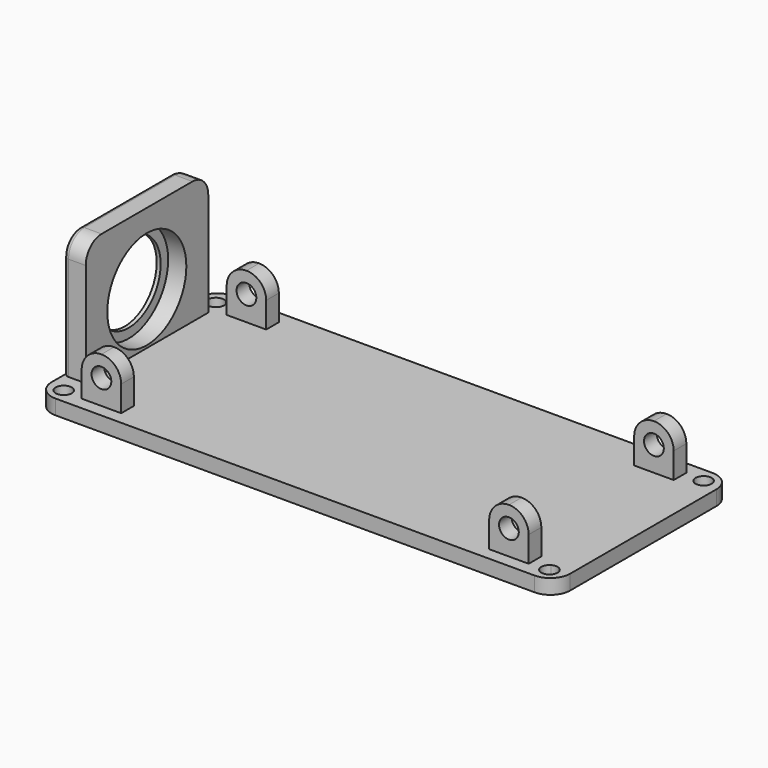
from build123d import *

# Parameters (mm, degrees)
F0_W      = 133.35
F0_H      = 57.15
F0_W_2    = 94.615
F0_H_2    = 4.064
F0_W_3    = 10.16
F0_H_3    = 42.545
F1_DEPTH  = 3.81
F2_W      = 5.6896
F2_H      = 39.37
F3_DEPTH  = 31.75
F4_R      = 5.08
F5_R      = 10.287
F6_DEPTH  = 25.4
F7_R      = 2.0701
F8_DEPTH  = 3.811
F9_R      = 5.08
F10_R     = 1.27
F11_R     = 12.7
F11_R_2   = 10.287
F12_DEPTH = 4.6736
F13_DEPTH = 15.494
F14_R     = 2.54
F15_DEPTH = 5.08
F16_R     = 2.54
F17_DEPTH = 25.4
F18_R     = 2.54
F19_DEPTH = 25.4
F20_R     = 2.54
F21_DEPTH = 25.4
F22_R     = 5.07999


# Not quite as in the source:
# - a fillet or chamfer is up to 0.001 mm smaller than in the source, because OpenCascade refuses the exact size


with BuildPart() as f1:
    # F0 (on Top) → F1 (new body)
    with BuildSketch(Plane.XY):
        Rectangle(F0_W, F0_H)
        Polygon((57.4675, -21.2725), (57.4675, -25.3365), (47.3075, -25.3365), (-47.3075, -25.3365), (-57.4675, -25.3365), (-57.4675, -21.2725), (-57.4675, 21.2725), (-57.4675, 25.3365), (-47.3075, 25.3365), (47.3075, 25.3365), (57.4675, 25.3365), (57.4675, 21.2725), align=None, mode=Mode.SUBTRACT)
        with Locations((0, 23.3045)):
            Rectangle(F0_W_2, F0_H_2)
        with Locations((-52.3875, 0)):
            Rectangle(F0_W_3, F0_H_3)
        with Locations((-52.3875, -23.3045)):
            Rectangle(F0_W_3, F0_H_2)
        with Locations((0, -23.3045)):
            Rectangle(F0_W_2, F0_H_2)
        Rectangle(F0_W_2, F0_H_3)
        with Locations((52.3875, 0)):
            Rectangle(F0_W_3, F0_H_3)
        with Locations((52.3875, -23.3045)):
            Rectangle(F0_W_3, F0_H_2)
        with Locations((52.3875, 23.3045)):
            Rectangle(F0_W_3, F0_H_2)
        with Locations((-52.3875, 23.3045)):
            Rectangle(F0_W_3, F0_H_2)
    extrude(amount=F1_DEPTH)

    # F2 (on face) → F3 (join)
    with BuildSketch(Plane.XY.offset(3.81)):
        with Locations((-63.8302, 0.0610498762)):
            Rectangle(F2_W, F2_H)
    extrude(amount=F3_DEPTH)

    # F4
    f4_edges = [f1.edges().sort_by_distance(p)[0] for p in [
        (-63.8302, 19.74605, 35.56),
        (-63.8302, -19.62395, 35.56),
    ]]
    fillet(f4_edges, radius=F4_R)

    # F5 (on face) → F6 (cut)
    with BuildSketch(Plane(origin=(-66.675, 0, 0), x_dir=(0, -1, 0), z_dir=(-1, 0, 0))):
        with Locations((0, 17.145)):
            Circle(F5_R)
    extrude(amount=-F6_DEPTH, mode=Mode.SUBTRACT)

    # F7 (on face) → F8 (cut, through all)
    with BuildSketch(Plane.XY.offset(3.81)):
        with Locations((-62.5474974513, 24.164236586)):
            Circle(F7_R)
        with Locations((62.3570047319, 24.7649991388)):
            Circle(F7_R)
        with BuildLine():
            ThreePointArc((64.4271047319, -24.7650008612), (64.1570098525, -23.7426038856), (63.4172061032, -22.987))
            Line((63.4172061032, -22.987), (61.2968033606, -22.987))
            ThreePointArc((61.2968033606, -22.987), (61.3346077563, -26.5650059818), (64.4271047319, -24.7650008612))
        make_face()
        with BuildLine():
            Line((61.2968033606, -22.987), (63.4172061032, -22.987))
            ThreePointArc((63.4172061032, -22.987), (62.3570047319, -22.6949008612), (61.2968033606, -22.987))
        make_face()
        with Locations((-62.5474974513, -24.7649997473)):
            Circle(F7_R)
    extrude(amount=-F8_DEPTH, mode=Mode.SUBTRACT)

    # F9
    f9_edges = [f1.edges().sort_by_distance(p)[0] for p in [
        (66.675, 28.575, 1.905),
        (-66.675, 28.575, 1.905),
        (-66.675, -28.575, 1.905),
        (66.675, -28.575, 1.905),
    ]]
    fillet(f9_edges, radius=F9_R)

    # F10
    f10_edges = [f1.edges().sort_by_distance(p)[0] for p in [
        (-66.675, 0.06105, 35.56),
    ]]
    fillet(f10_edges, radius=F10_R)

    # F11 (on face) → F12 (cut)
    with BuildSketch(Plane.YZ.offset(-60.9854)):
        with Locations((0, 17.145)):
            Circle(F11_R)
        with Locations((0, 17.145)):
            Circle(F11_R_2, mode=Mode.SUBTRACT)
    extrude(amount=-F12_DEPTH, mode=Mode.SUBTRACT)

    # F0 (on Top) → F13 (join)
    with BuildSketch(Plane.XY):
        with Locations((52.3875, 23.3045)):
            Rectangle(F0_W_3, F0_H_2)
        with Locations((52.3875, -23.3045)):
            Rectangle(F0_W_3, F0_H_2)
        with Locations((-52.3875, 23.3045)):
            Rectangle(F0_W_3, F0_H_2)
        with Locations((-52.3875, -23.3045)):
            Rectangle(F0_W_3, F0_H_2)
    extrude(amount=F13_DEPTH)

    # F14 (on face) → F15 (cut)
    with BuildSketch(Plane(origin=(0, 25.3365, 0), x_dir=(-1, 0, 0), z_dir=(0, 1, 0))):
        with Locations((52.3874983191, 10.1600000635)):
            Circle(F14_R)
    extrude(amount=-F15_DEPTH, mode=Mode.SUBTRACT)

    # F16 (on face) → F17 (cut)
    with BuildSketch(Plane.XZ.offset(25.3365)):
        with Locations((52.3875, 10.16)):
            Circle(F16_R)
    extrude(amount=-F17_DEPTH, mode=Mode.SUBTRACT)

    # F18 (on face) → F19 (cut)
    with BuildSketch(Plane.XZ.offset(-21.2725)):
        with Locations((52.3875, 10.16)):
            Circle(F18_R)
    extrude(amount=-F19_DEPTH, mode=Mode.SUBTRACT)

    # F20 (on face) → F21 (cut)
    with BuildSketch(Plane.XZ.offset(25.3365)):
        with Locations((-52.3875, 10.16)):
            Circle(F20_R)
    extrude(amount=-F21_DEPTH, mode=Mode.SUBTRACT)

    # F22 (radius 5.08 in the source; OpenCascade refuses exactly that, so slightly less here)
    f22_edges = [f1.edges().sort_by_distance(p)[0] for p in [
        (-47.3075, -23.3045, 15.494),
        (-57.4675, -23.3045, 15.494),
        (-57.4675, 23.3045, 15.494),
        (-47.3075, 23.3045, 15.494),
        (47.3075, 23.3045, 15.494),
        (47.3075, -23.3045, 15.494),
        (57.4675, -23.3045, 15.494),
        (57.4675, 23.3045, 15.494),
    ]]
    fillet(f22_edges, radius=F22_R)


solid = f1.part
